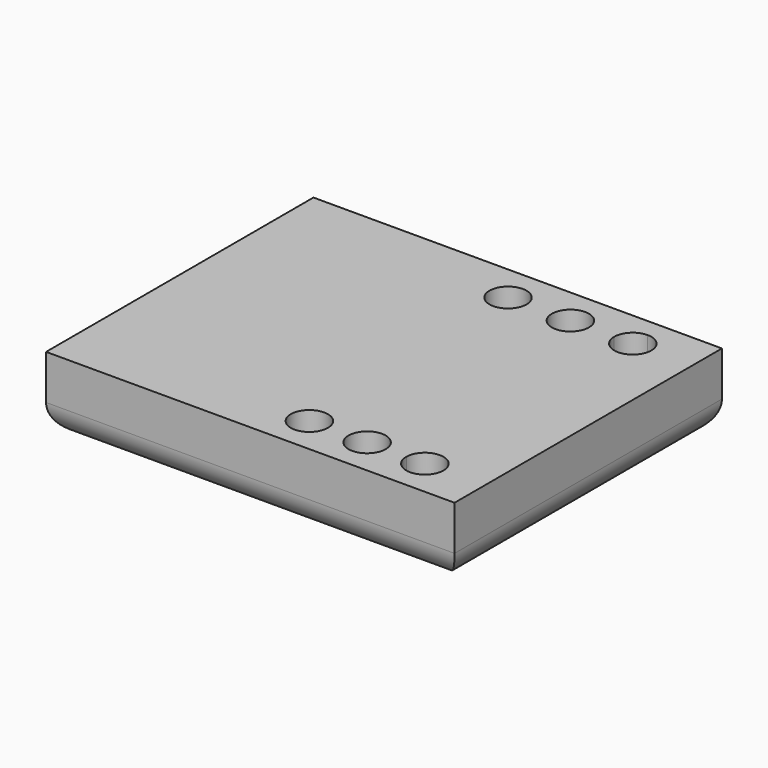
from build123d import *

# Parameters (mm, degrees)
F0_R        = 3.175
F1_DEPTH    = 12.7
F2_T1_DEPTH = 95.25
F2_T3_DEPTH = 82.55


# Not quite as in the source:
# - a fillet or chamfer that OpenCascade refuses, or shapes differently, is made with other operations: its cross-section is extruded or revolved along the edge and cut away or added


with BuildPart() as f1:
    # F0 (on Top) → F1 (new body)
    with BuildSketch(Plane.XY):
        with BuildLine():
            Line((23.8110734844, 40.5260987967), (-35.8789265156, 40.5260987967))
            Line((-35.8789265156, 40.5260987967), (-35.8789265156, -16.6239012033))
            Line((-35.8789265156, -16.6239012033), (23.8110734844, -16.6239012033))
            Line((23.8110734844, -16.6239012033), (23.8110734844, -13.4489012033))
            ThreePointArc((23.8110734844, -13.4489012033), (21.5660094542, -12.5189652335), (20.6360734844, -10.2739012033))
            ThreePointArc((20.6360734844, -10.2739012033), (23.8110734844, -7.0989012033), (26.9860734844, -10.2739012033))
            Line((26.9860734844, -10.2739012033), (33.9710734844, -10.2739012033))
            Line((33.9710734844, -10.2739012033), (33.9710734844, 34.1760987967))
            Line((33.9710734844, 34.1760987967), (26.9860734844, 34.1760987967))
            ThreePointArc((26.9860734844, 34.1760987967), (23.8110734844, 31.0010987967), (20.6360734844, 34.1760987967))
            ThreePointArc((20.6360734844, 34.1760987967), (21.5660094542, 36.421162827), (23.8110734844, 37.3510987967))
            Line((23.8110734844, 37.3510987967), (23.8110734844, 40.5260987967))
        make_face()
        with Locations((4.0669361824, -10.2739012033)):
            Circle(F0_R, mode=Mode.SUBTRACT)
        with BuildLine():
            ThreePointArc((10.7640048334, -10.2739012033), (13.9390048334, -7.0989012033), (17.1140048334, -10.2739012033))
            ThreePointArc((17.1140048334, -10.2739012033), (13.9390048334, -13.4489012033), (10.7640048334, -10.2739012033))
        make_face(mode=Mode.SUBTRACT)
        with Locations((2.4716164917, 34.1760987967)):
            Circle(F0_R, mode=Mode.SUBTRACT)
        with BuildLine():
            ThreePointArc((9.966344988, 34.1760987967), (13.141344988, 37.3510987967), (16.316344988, 34.1760987967))
            ThreePointArc((16.316344988, 34.1760987967), (13.141344988, 31.0010987967), (9.966344988, 34.1760987967))
        make_face(mode=Mode.SUBTRACT)
        with BuildLine():
            Line((33.9710734844, 40.5260987967), (23.8110734844, 40.5260987967))
            Line((23.8110734844, 40.5260987967), (23.8110734844, 37.3510987967))
            ThreePointArc((23.8110734844, 37.3510987967), (26.0561375147, 36.421162827), (26.9860734844, 34.1760987967))
            Line((26.9860734844, 34.1760987967), (33.9710734844, 34.1760987967))
            Line((33.9710734844, 34.1760987967), (33.9710734844, 40.5260987967))
        make_face()
        with BuildLine():
            Line((23.8110734844, -13.4489012033), (23.8110734844, -16.6239012033))
            Line((23.8110734844, -16.6239012033), (33.9710734844, -16.6239012033))
            Line((33.9710734844, -16.6239012033), (33.9710734844, -10.2739012033))
            Line((33.9710734844, -10.2739012033), (26.9860734844, -10.2739012033))
            ThreePointArc((26.9860734844, -10.2739012033), (26.0561375147, -12.5189652335), (23.8110734844, -13.4489012033))
        make_face()
    extrude(amount=F1_DEPTH)

    # F2: fillet of radius 5.08 on 4 edges, made by hand

    # F2_s2 → F2_t1 (cut)
    with BuildSketch(Plane.YZ.offset(-48.5789265156)):
        with BuildLine():
            ThreePointArc((-16.6239012033, 5.08), (-15.1360036517, 1.4878975516), (-11.5439012033, 0))
            Line((-11.5439012033, 0), (-16.6239012033, 0))
            Line((-16.6239012033, 0), (-16.6239012033, 5.08))
        make_face()
        with BuildLine():
            ThreePointArc((40.5260987967, 5.08), (39.0382012452, 1.4878975516), (35.4460987967, 0))
            Line((35.4460987967, 0), (40.5260987967, 0))
            Line((40.5260987967, 0), (40.5260987967, 5.08))
        make_face()
    extrude(amount=F2_T1_DEPTH, mode=Mode.SUBTRACT)

    # F2_s4 → F2_t3 (cut)
    with BuildSketch(Plane.XZ.offset(-53.2260987967)):
        with BuildLine():
            ThreePointArc((33.9710734844, 5.08), (32.4831759328, 1.4878975516), (28.8910734844, 0))
            Line((28.8910734844, 0), (33.9710734844, 0))
            Line((33.9710734844, 0), (33.9710734844, 5.08))
        make_face()
        with BuildLine():
            ThreePointArc((-35.8789265156, 5.08), (-34.391028964, 1.4878975516), (-30.7989265156, 0))
            Line((-30.7989265156, 0), (-35.8789265156, 0))
            Line((-35.8789265156, 0), (-35.8789265156, 5.08))
        make_face()
    extrude(amount=F2_T3_DEPTH, mode=Mode.SUBTRACT)


solid = f1.part
